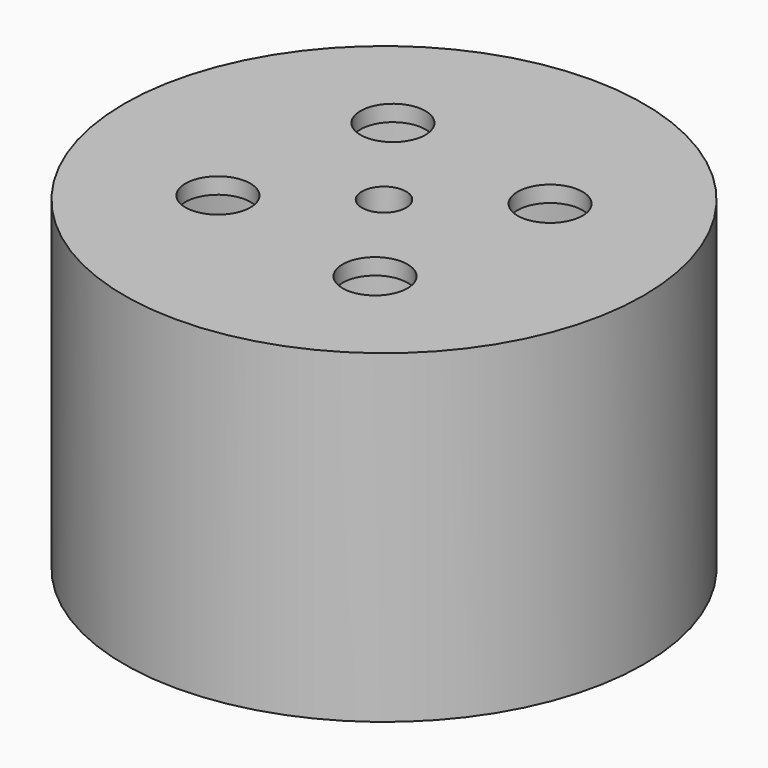
from build123d import *

# Parameters (mm, degrees)
F0_R      = 40
F0_R_2    = 2
F0_R_3    = 3.4
F1_DEPTH  = 50
F2_R      = 7.220544461
F3_DEPTH  = 45
F4_R      = 5
F5_DEPTH  = 10
F6_T      = 2.5
F5_FACE_R = 5
F7_DEPTH  = 15


# Not quite as in the source:
# - a shell that OpenCascade refuses in one call is made with other operations: the cavity is built on its own and cut out


with BuildPart() as f1:
    # F0 (on Top) → F1 (new body)
    with BuildSketch(Plane.XY):
        Circle(F0_R)
        with Locations((-16.2671870079, -11.6352321356)):
            Circle(F0_R_2, mode=Mode.SUBTRACT)
        with Locations((11.6352321356, -16.2671870079)):
            Circle(F0_R_2, mode=Mode.SUBTRACT)
        with Locations((-11.6352321356, 16.2671870079)):
            Circle(F0_R_2, mode=Mode.SUBTRACT)
        Circle(F0_R_3, mode=Mode.SUBTRACT)
        with Locations((16.2671870079, 11.6352321356)):
            Circle(F0_R_2, mode=Mode.SUBTRACT)
    extrude(amount=F1_DEPTH)

    # F2 (on Top) → F3 (cut)
    with BuildSketch(Plane.XY):
        Circle(F2_R)
    extrude(amount=F3_DEPTH, mode=Mode.SUBTRACT)

    # F6: shell of thickness 2.5, made by hand


with BuildPart() as f5:
    # F4 (on face) → F5 (new body)
    with BuildSketch(Plane.XY.offset(50)):
        with Locations((-11.6352321356, 16.2671870079)):
            Circle(F4_R)
    extrude(amount=-F5_DEPTH)


with BuildPart() as f5b:
    # F4 (on face) → F5, piece 2 (new body)
    with BuildSketch(Plane.XY.offset(50)):
        with Locations((16.2671870079, 11.6352321356)):
            Circle(F4_R)
    extrude(amount=-F5_DEPTH)


with BuildPart() as f5c:
    # F4 (on face) → F5, piece 3 (new body)
    with BuildSketch(Plane.XY.offset(50)):
        with Locations((11.6352321356, -16.2671870079)):
            Circle(F4_R)
    extrude(amount=-F5_DEPTH)


with BuildPart() as f5d:
    # F4 (on face) → F5, piece 4 (new body)
    with BuildSketch(Plane.XY.offset(50)):
        with Locations((-16.2671870079, -11.6352321356)):
            Circle(F4_R)
    extrude(amount=-F5_DEPTH)


with BuildPart() as f6_core1:
    # F6_t2: copy of F1
    add(f1.part)

    # the walls: a layer under each face that stays
    f6_faces = [f6_core1.faces().sort_by_distance(p)[0] for p in [
        (-40, 0, 25),
        (-26.6666666667, -26.6666666667, 50),
        (-18.2671870079, -11.6352321356, 25),
        (9.6352321356, -16.2671870079, 25),
        (-7.220544461, 0, 22.5),
        (-13.6352321356, 16.2671870079, 25),
        (14.2671870079, 11.6352321356, 25),
        (-3.4, 0, 47.5),
        (-4.8136963073, -4.8136963073, 45),
    ]]
    thicken(f6_faces, amount=-F6_T, mode=Mode.SUBTRACT)

    # F6_s3 → F6_t4 (revolve, cut)
    with BuildSketch(Plane.XZ):
        Polygon((7.195544461, 44.975), (9.720544461, 45), (9.720544461, 47.5), (7.220544461, 47.5), align=None)
    revolve(axis=Axis((0, 0, 45), (0, 0, 1)), mode=Mode.SUBTRACT)


with BuildPart() as f1_1:
    add(f1.part)

    # what is left inside the walls is the cavity
    f6_cavity = [f6_core1.part.solids().sort_by_distance(p)[0] for p in [
        (-37.475, 0, 31.666667),
    ]]
    add(f6_cavity, mode=Mode.SUBTRACT)


with BuildPart() as f7_tool:
    # F5_face (on face) → F7 (new body)
    with BuildSketch(Plane(origin=(-11.6352321356, 16.2671870079, 50), x_dir=(1, 0, 0), z_dir=(0, 0, 1))):
        Circle(F5_FACE_R)
        with Locations((23.2704642711, -32.5343740159)):
            Circle(F5_FACE_R)
        with Locations((27.9024191435, -4.6319548724)):
            Circle(F5_FACE_R)
        with Locations((-4.6319548724, -27.9024191435)):
            Circle(F5_FACE_R)
    extrude(amount=-F7_DEPTH)


with BuildPart() as f1_2:
    add(f1_1.part)

    # F7: cut by f7_tool
    add(f7_tool.part, mode=Mode.SUBTRACT)


with BuildPart() as f5_1:
    add(f5.part)

    # F7: cut by f7_tool
    add(f7_tool.part, mode=Mode.SUBTRACT)


with BuildPart() as f5b_1:
    add(f5b.part)

    # F7: cut by f7_tool
    add(f7_tool.part, mode=Mode.SUBTRACT)


with BuildPart() as f5c_1:
    add(f5c.part)

    # F7: cut by f7_tool
    add(f7_tool.part, mode=Mode.SUBTRACT)


with BuildPart() as f5d_1:
    add(f5d.part)

    # F7: cut by f7_tool
    add(f7_tool.part, mode=Mode.SUBTRACT)


solid = f1_2.part
